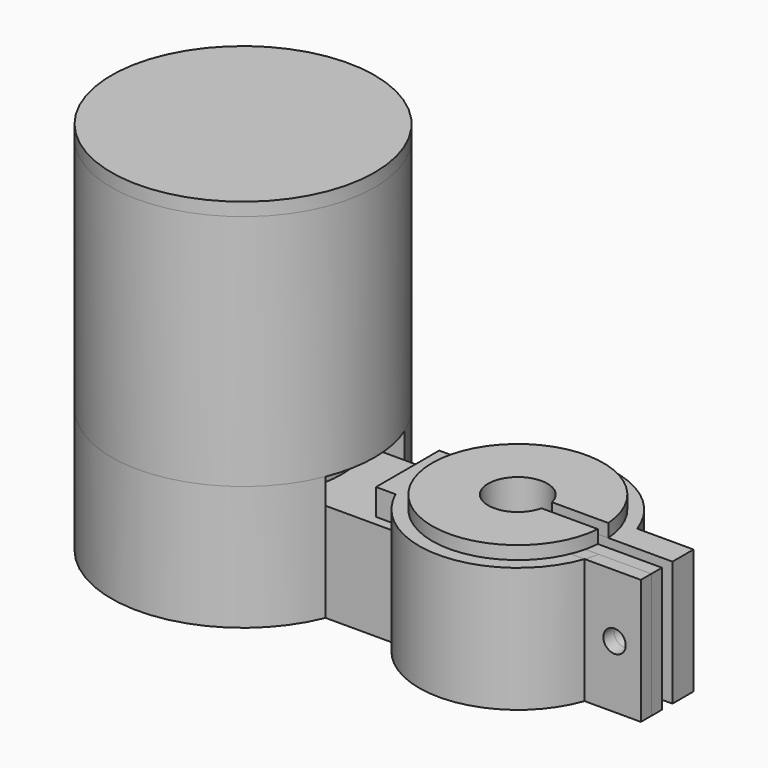
from build123d import *
from build123d import SkipClean  # not in build123d's __all__

# Parameters (mm, degrees)
F1_DEPTH      = 4
F2_DEPTH      = 15
F3_DEPTH      = 30
F3_DEPTH_BACK = 15
F4_R          = 1.7
F5_DEPTH      = 0.5
F6_DEPTH      = 6
F8_DEPTH      = 19
F9_DEPTH      = 2
F11_DEPTH     = 2
F12_R         = 1.7
F13_DEPTH     = 2
F15_R         = 2.5
F16_DEPTH     = 2.5
F15_R_2       = 20
F15_R_3       = 15
F17_DEPTH     = 36.1
F18_DEPTH     = 2
F20_DEPTH     = 18.9


with BuildPart() as f1:
    # F0 (on Top) → F1 (new body)
    with BuildSketch(Plane.XY):
        with BuildLine():
            ThreePointArc((28, -6), (26.7477270849, 0), (28, 6))
            Line((28, 6), (25, 6))
            Line((25, 6), (25, 0))
            Line((25, 0), (25, -6))
            Line((25, -6), (28, -6))
        make_face()
        with BuildLine():
            ThreePointArc((52.702178235, -1), (30.7477270849, 0), (52.702178235, 1))
            Line((52.702178235, 1), (56.4446655416, 1))
            Line((56.4446655416, 1), (64.4446655416, 1))
            Line((64.4446655416, 1), (64.4446655416, 3))
            Line((64.4446655416, 3), (56.4446655416, 3))
            ThreePointArc((56.4446655416, 3), (44.1540904281, 14.805722389), (28.7573460281, 7.5))
            ThreePointArc((28.7573460281, 7.5), (28.3576521505, 6.7606133784), (28, 6))
            ThreePointArc((28, 6), (26.7477270849, 0), (28, -6))
            ThreePointArc((28, -6), (28.3576521505, -6.7606133784), (28.7573460281, -7.5))
            ThreePointArc((28.7573460281, -7.5), (44.1540904281, -14.805722389), (56.4446655416, -3))
            Line((56.4446655416, -3), (64.4446655416, -3))
            Line((64.4446655416, -3), (64.4446655416, -1))
            Line((64.4446655416, -1), (56.4446655416, -1))
            Line((56.4446655416, -1), (52.702178235, -1))
        make_face()
    extrude(amount=F1_DEPTH)

    # F0 (on Top) → F2 (join)
    with BuildSketch(Plane.XY):
        with BuildLine():
            ThreePointArc((52.702178235, -1), (30.7477270849, 0), (52.702178235, 1))
            Line((52.702178235, 1), (56.4446655416, 1))
            Line((56.4446655416, 1), (64.4446655416, 1))
            Line((64.4446655416, 1), (64.4446655416, 3))
            Line((64.4446655416, 3), (56.4446655416, 3))
            ThreePointArc((56.4446655416, 3), (44.1540904281, 14.805722389), (28.7573460281, 7.5))
            ThreePointArc((28.7573460281, 7.5), (28.3576521505, 6.7606133784), (28, 6))
            ThreePointArc((28, 6), (26.7477270849, 0), (28, -6))
            ThreePointArc((28, -6), (28.3576521505, -6.7606133784), (28.7573460281, -7.5))
            ThreePointArc((28.7573460281, -7.5), (44.1540904281, -14.805722389), (56.4446655416, -3))
            Line((56.4446655416, -3), (64.4446655416, -3))
            Line((64.4446655416, -3), (64.4446655416, -1))
            Line((64.4446655416, -1), (56.4446655416, -1))
            Line((56.4446655416, -1), (52.702178235, -1))
        make_face()
        with BuildLine():
            ThreePointArc((28, -6), (26.7477270849, 0), (28, 6))
            Line((28, 6), (25, 6))
            Line((25, 6), (25, 0))
            Line((25, 0), (25, -6))
            Line((25, -6), (28, -6))
        make_face()
        with BuildLine():
            ThreePointArc((28, 6), (28.3576521505, 6.7606133784), (28.7573460281, 7.5))
            Line((28.7573460281, 7.5), (12.9903810568, 7.5))
            ThreePointArc((12.9903810568, 7.5), (14.4888873943, 3.8822856765), (15, 0))
            ThreePointArc((15, 0), (14.4888873943, -3.8822856765), (12.9903810568, -7.5))
            Line((12.9903810568, -7.5), (28.7573460281, -7.5))
            ThreePointArc((28.7573460281, -7.5), (28.3576521505, -6.7606133784), (28, -6))
            Line((28, -6), (25, -6))
            Line((25, -6), (25, 0))
            Line((25, 0), (25, 6))
            Line((25, 6), (28, 6))
        make_face()
    extrude(amount=-F2_DEPTH)

    # F0 (on Top) → F3 (join, two sides)
    with BuildSketch(Plane.XY) as f3_sk:
        with BuildLine():
            ThreePointArc((15, 0), (14.4888873943, 3.8822856765), (12.9903810568, 7.5))
            ThreePointArc((12.9903810568, 7.5), (-15, 0), (12.9903810568, -7.5))
            ThreePointArc((12.9903810568, -7.5), (14.4888873943, -3.8822856765), (15, 0))
        make_face()
    extrude(amount=F3_DEPTH)
    extrude(f3_sk.sketch, amount=-F3_DEPTH_BACK)

    # F4 (on face) → F5 (cut)
    with BuildSketch(Plane(origin=(0, 3, 0), x_dir=(-1, 0, 0), z_dir=(0, 1, 0))):
        Polygon((-63.2446655416, -7.1165807537), (-60.4446655416, -8.7331615075), (-57.6446655416, -7.1165807537), (-57.6446655416, -3.8834192463), (-60.4446655416, -2.2668384925), (-63.2446655416, -3.8834192463), align=None)
        with Locations((-60.4446655416, -5.5)):
            Circle(F4_R, mode=Mode.SUBTRACT)
    extrude(amount=-F5_DEPTH, mode=Mode.SUBTRACT)

    # F6 (cut, through all): a face of the model
    f6_faces = [f1.faces().sort_by_distance(p)[0] for p in [
        (60.4446655416, 3, -5.5),
    ]]
    extrude(f6_faces, amount=-F6_DEPTH, mode=Mode.SUBTRACT)

    # F10 (on face) → F11 (join)
    with BuildSketch(Plane(origin=(0, 3, 0), x_dir=(-1, 0, 0), z_dir=(0, 1, 0))):
        Polygon((-64.4446655416, -15), (-56.4446655416, -15), (-52.5044240057, -15), (-52.5044240057, 4), (-56.4446655416, 4), (-64.4446655416, 4), align=None)
        Polygon((-63.2446655416, -7.1165807537), (-63.2446655416, -3.8834192463), (-60.4446655416, -2.2668384925), (-57.6446655416, -3.8834192463), (-57.6446655416, -7.1165807537), (-60.4446655416, -8.7331615075), align=None, mode=Mode.SUBTRACT)
    extrude(amount=F11_DEPTH)

    # F12 (on face) → F13 (join)
    with BuildSketch(Plane.XZ.offset(3)):
        Polygon((64.4446655416, 4), (56.4446655416, 4), (52.1536841989, 4), (52.1536841989, -15), (56.4446655416, -15), (64.4446655416, -15), align=None)
        with Locations((60.4446655416, -5.5)):
            Circle(F12_R, mode=Mode.SUBTRACT)
    with SkipClean():  # cleaning this boolean's faces spoils the solid; the shape is the same uncleaned
        extrude(amount=F13_DEPTH)


with BuildPart() as f8:
    # F7 (on face) → F8 (new body, through all)
    with BuildSketch(Plane.XY.offset(4)):
        with BuildLine():
            Line((46.1352092786, 1), (52.702178235, 1))
            ThreePointArc((52.702178235, 1), (30.7477270849, 0), (52.702178235, -1))
            Line((52.702178235, -1), (46.1352092786, -1))
            ThreePointArc((46.1352092786, -1), (37.2477270849, 0), (46.1352092786, 1))
        make_face()
    extrude(amount=-F8_DEPTH)

    # F7 (on face) → F9 (join)
    with BuildSketch(Plane.XY.offset(4)):
        with BuildLine():
            Line((46.1352092786, 1), (52.702178235, 1))
            ThreePointArc((52.702178235, 1), (30.7477270849, 0), (52.702178235, -1))
            Line((52.702178235, -1), (46.1352092786, -1))
            ThreePointArc((46.1352092786, -1), (37.2477270849, 0), (46.1352092786, 1))
        make_face()
        with BuildLine():
            ThreePointArc((52.702178235, -1), (30.7477270849, 0), (52.702178235, 1))
            Line((52.702178235, 1), (54.7092084817, 1))
            ThreePointArc((54.7092084817, 1), (28.7477270849, 0), (54.7092084817, -1))
            Line((54.7092084817, -1), (52.702178235, -1))
        make_face()
    extrude(amount=F9_DEPTH)


with BuildPart() as f16:
    # F15 (on offset) → F16 (new body)
    with BuildSketch(Plane.XY.offset(40)):
        Circle(F15_R)
    extrude(amount=-F16_DEPTH)



with BuildPart() as f17:
    # F15 (on offset) → F17 (new body)
    with BuildSketch(Plane.XY.offset(40)):
        Circle(F15_R_2)
        Circle(F15_R_3, mode=Mode.SUBTRACT)
    extrude(amount=-F17_DEPTH)


with BuildPart() as f16_1:
    add(f16.part, clean=False)

    add(f17.part)  # F18 merges F17
    # F15 (on offset) → F18 (join)
    with BuildSketch(Plane.XY.offset(40)):
        Circle(F15_R_2)
        Circle(F15_R_3, mode=Mode.SUBTRACT)
        Circle(F15_R_3)
        Circle(F15_R, mode=Mode.SUBTRACT)
        Circle(F15_R)
    extrude(amount=F18_DEPTH)

    # F19 (on face) → F20 (join, through all)
    with BuildSketch(Plane(origin=(0, 0, 3.9), x_dir=(1, 0, 0), z_dir=(0, 0, -1))):
        with BuildLine():
            ThreePointArc((12.9903810568, -7.5), (-15, 0), (12.9903810568, 7.5))
            Line((12.9903810568, 7.5), (18.5404962177, 7.5))
            ThreePointArc((18.5404962177, 7.5), (-20, 0), (18.5404962177, -7.5))
            Line((18.5404962177, -7.5), (12.9903810568, -7.5))
        make_face()
    extrude(amount=F20_DEPTH)


solid = Compound([f1.part, f8.part, f16_1.part])
